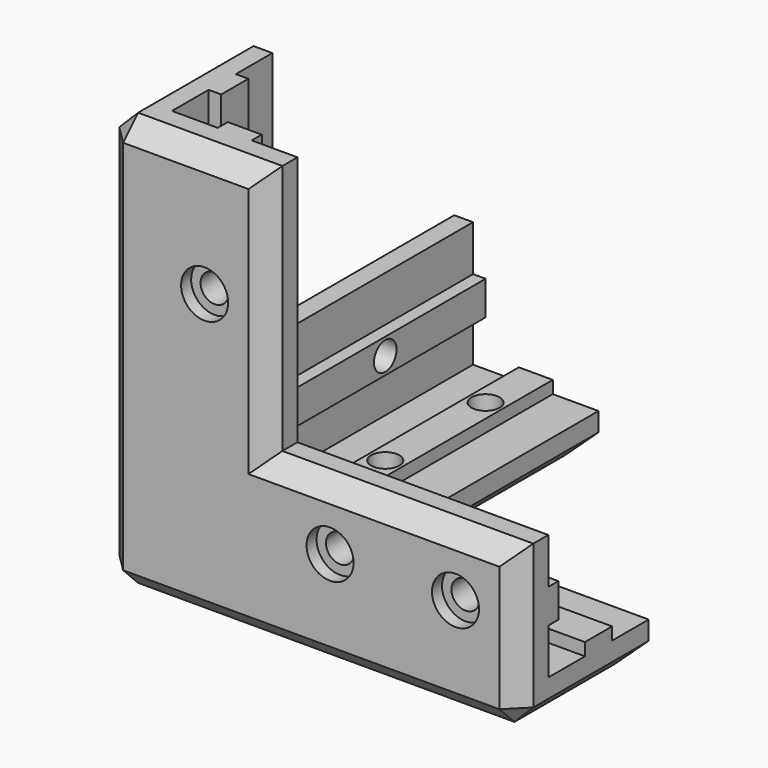
from build123d import *

# Parameters (mm, degrees)
F1_DEPTH  = 6
F3_DEPTH  = 20
F5_DEPTH  = 40
F7_DEPTH  = 60
F9_DEPTH  = 2
F11_DEPTH = 2
F13_DEPTH = 2
F14_R     = 2.25
F15_DEPTH = 8
F16_R     = 2.25
F17_DEPTH = 8
F18_R     = 2.25
F19_DEPTH = 8
F20_R     = 3.75
F21_DEPTH = 2
F22_R     = 3.75
F23_DEPTH = 2
F24_R     = 3.75
F25_DEPTH = 2
F26_SIZE  = 3


with BuildPart() as f1:
    # F0 (on Top) → F1 (new body)
    with BuildSketch(Plane.XY):
        Polygon((0, 66), (0, 0), (66, 0), (66, 26), (26, 26), (26, 66), align=None)
    extrude(amount=F1_DEPTH)

    # F2 (on face) → F3 (join)
    with BuildSketch(Plane.XY.offset(6)):
        Polygon((6, 66), (0, 66), (0, 0), (66, 0), (66, 6), (6, 6), align=None)
    extrude(amount=F3_DEPTH)

    # F4 (on face) → F5 (join)
    with BuildSketch(Plane.XY.offset(26)):
        Polygon((6, 6), (6, 26), (0, 26), (0, 0), (26, 0), (26, 6), align=None)
    extrude(amount=F5_DEPTH)

    # F6 (on face) → F7 (join)
    with BuildSketch(Plane.XY.offset(6)):
        Polygon((13.29, 6), (16, 6), (18.71, 6), (18.71, 8), (13.29, 8), align=None)
        Polygon((6, 18.71), (6, 16), (6, 13.29), (8, 13.29), (8, 18.71), align=None)
    extrude(amount=F7_DEPTH)

    # F8 (on face) → F9 (join)
    with BuildSketch(Plane.XY.offset(6)):
        Polygon((66, 13.29), (66, 16), (66, 18.71), (26, 18.71), (26, 13.29), align=None)
        Polygon((18.71, 66), (16, 66), (13.29, 66), (13.29, 26), (18.71, 26), align=None)
    extrude(amount=F9_DEPTH)

    # F10 (on face) → F11 (join)
    with BuildSketch(Plane(origin=(0, 6, 0), x_dir=(-1, 0, 0), z_dir=(0, 1, 0))):
        Polygon((-66, 18.71), (-66, 16), (-66, 13.29), (-26, 13.29), (-26, 16), (-26, 18.71), align=None)
    extrude(amount=F11_DEPTH)

    # F12 (on face) → F13 (join)
    with BuildSketch(Plane.YZ.offset(6)):
        Polygon((66, 13.29), (66, 16), (66, 18.71), (26, 18.71), (26, 13.29), align=None)
    extrude(amount=F13_DEPTH)

    # F14 (on face) → F15 (cut, through all)
    with BuildSketch(Plane.XZ):
        with Locations((56, 16)):
            Circle(F14_R)
        with Locations((16, 46)):
            Circle(F14_R)
        with Locations((36, 16)):
            Circle(F14_R)
    extrude(amount=-F15_DEPTH, mode=Mode.SUBTRACT)

    # F16 (on face) → F17 (cut, through all)
    with BuildSketch(Plane(origin=(0, 0, 0), x_dir=(0, -1, 0), z_dir=(-1, 0, 0))):
        with Locations((-16, 56)):
            Circle(F16_R)
        with Locations((-46, 16)):
            Circle(F16_R)
        with Locations((-16, 36)):
            Circle(F16_R)
    extrude(amount=-F17_DEPTH, mode=Mode.SUBTRACT)

    # F18 (on face) → F19 (cut, through all)
    with BuildSketch(Plane(origin=(0, 0, 0), x_dir=(1, 0, 0), z_dir=(0, 0, -1))):
        with Locations((46, -16)):
            Circle(F18_R)
        with Locations((16, -56)):
            Circle(F18_R)
        with Locations((16, -36)):
            Circle(F18_R)
    extrude(amount=-F19_DEPTH, mode=Mode.SUBTRACT)

    # F20 (on face) → F21 (cut)
    with BuildSketch(Plane.XZ):
        with Locations((16, 46)):
            Circle(F20_R)
        with Locations((36, 16)):
            Circle(F20_R)
        with Locations((56, 16)):
            Circle(F20_R)
    extrude(amount=-F21_DEPTH, mode=Mode.SUBTRACT)

    # F22 (on face) → F23 (cut)
    with BuildSketch(Plane(origin=(0, 0, 0), x_dir=(0, -1, 0), z_dir=(-1, 0, 0))):
        with Locations((-16, 56)):
            Circle(F22_R)
        with Locations((-46, 16)):
            Circle(F22_R)
        with Locations((-16, 36)):
            Circle(F22_R)
    extrude(amount=-F23_DEPTH, mode=Mode.SUBTRACT)

    # F24 (on face) → F25 (cut)
    with BuildSketch(Plane(origin=(0, 0, 0), x_dir=(1, 0, 0), z_dir=(0, 0, -1))):
        with Locations((16, -56)):
            Circle(F24_R)
        with Locations((46, -16)):
            Circle(F24_R)
        with Locations((16, -36)):
            Circle(F24_R)
    extrude(amount=-F25_DEPTH, mode=Mode.SUBTRACT)

    # F26
    f26_edges = [f1.edges().sort_by_distance(p)[0] for p in [
        (33, 0, 0),
        (0, 33, 0),
        (0, 0, 33),
        (0, 26, 46),
        (0, 46, 26),
        (26, 0, 46),
        (46, 0, 26),
        (0, 13, 66),
        (13, 0, 66),
        (0, 66, 13),
        (13, 66, 0),
        (66, 0, 13),
        (66, 13, 0),
        (46, 26, 0),
        (26, 46, 0),
    ]]
    chamfer(f26_edges, length=F26_SIZE)


solid = f1.part
